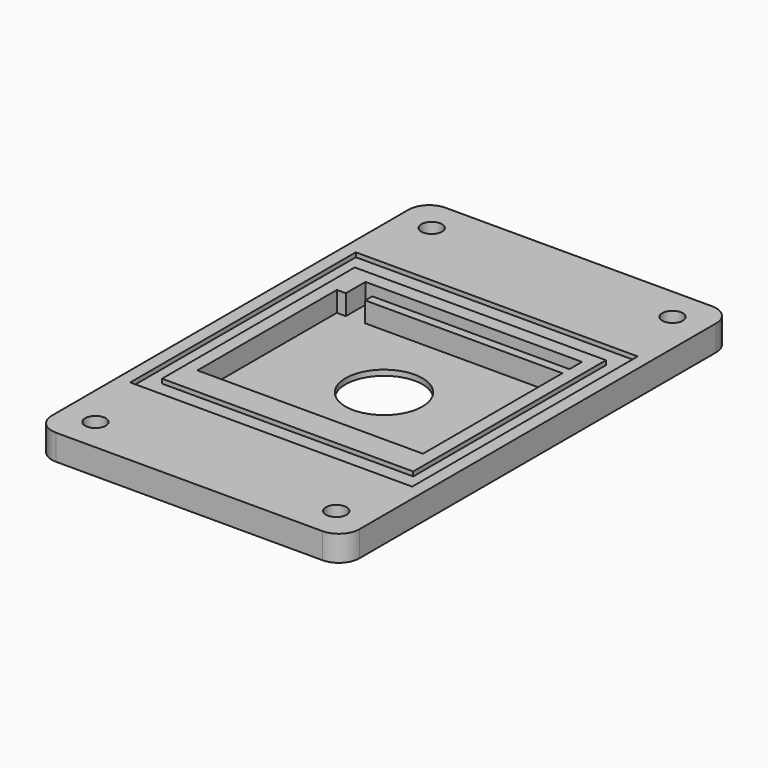
from build123d import *

# Parameters (mm, degrees)
F0_W     = 76.2
F0_H     = 120.65
F0_R     = 2.5527
F1_DEPTH = 6.35
F2_R     = 9.525
F3_DEPTH = 6.35
F2_W     = 55.88
F2_H     = 43.18
F4_DEPTH = 5
F5_R     = 5.08
F6_W     = 69.85
F6_H     = 69.85
F6_W_2   = 62.23
F6_H_2   = 59.69
F7_DEPTH = 1.08458
F9_DEPTH = 5


# Not quite as in the source:
# - a length typed as a fraction of an inch, garbled in the dataset ("3 / 203.2 mm" for 3/8 in), is restored


with BuildPart() as f1:
    # F0 (on Top) → F1 (new body)
    with BuildSketch(Plane.XY):
        Rectangle(F0_W, F0_H)
        with Locations((-29.8323, -52.0573)):
            Circle(F0_R, mode=Mode.SUBTRACT)
        with Locations((29.8323, -52.0573)):
            Circle(F0_R, mode=Mode.SUBTRACT)
        with Locations((-29.8323, 52.0573)):
            Circle(F0_R, mode=Mode.SUBTRACT)
        with Locations((29.8323, 52.0573)):
            Circle(F0_R, mode=Mode.SUBTRACT)
    extrude(amount=F1_DEPTH)

    # F2 (on face) → F3 (cut)
    with BuildSketch(Plane.XY.offset(6.35)):
        Circle(F2_R)
    extrude(amount=-F3_DEPTH, mode=Mode.SUBTRACT)

    # F2 (on face) → F4 (cut)
    with BuildSketch(Plane.XY.offset(6.35)):
        with Locations((0, -1.27)):
            Rectangle(F2_W, F2_H)
        Circle(F2_R, mode=Mode.SUBTRACT)
    extrude(amount=-F4_DEPTH, mode=Mode.SUBTRACT)

    # F5
    f5_edges = [f1.edges().sort_by_distance(p)[0] for p in [
        (38.1, -60.325, 3.175),
        (38.1, 60.325, 3.175),
        (-38.1, 60.325, 3.175),
        (-38.1, -60.325, 3.175),
    ]]
    fillet(f5_edges, radius=F5_R)

    # F6 (on face) → F7 (cut)
    with BuildSketch(Plane.XY.offset(6.35)):
        Rectangle(F6_W, F6_H)
        Rectangle(F6_W_2, F6_H_2, mode=Mode.SUBTRACT)
    extrude(amount=-F7_DEPTH, mode=Mode.SUBTRACT)

    # F8 (on face) → F9 (cut)
    with BuildSketch(Plane.XY.offset(6.35)):
        Polygon((-25.7090758532, 20.32), (-20.905200392, 20.32), (-20.905200392, 22.5038137287), (27.94, 22.5038137287), (27.94, 26.3926647604), (-25.7090758532, 26.3926647604), align=None)
    extrude(amount=-F9_DEPTH, mode=Mode.SUBTRACT)


solid = f1.part
